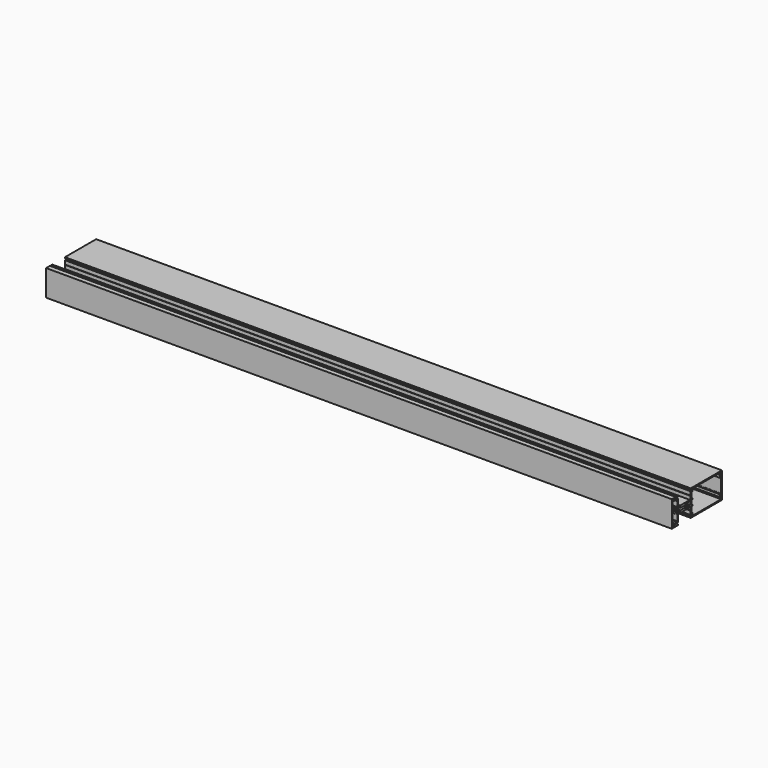
from build123d import *

# Parameters (mm, degrees)
F1_DEPTH = 1524
F2_DEPTH = 127


# Not quite as in the source:
# - ends of sketch curves that miss each other by under 0.0002 mm in the source are joined


with BuildPart() as f1:
    # F0 (on Right) → F1 (new body)
    with BuildSketch(Plane.YZ):
        with BuildLine():
            Line((-18.542, -31.745936), (76.2, -31.745936))
            Line((76.2, -31.745936), (76.2, -31.263336))
            Line((76.2, -31.263336), (76.2, 31.754064))
            Line((76.2, 31.754064), (-18.542, 31.754064))
            ThreePointArc((-18.542, 31.754064), (-18.9012102448, 31.6052742448), (-19.05, 31.246064))
            Line((-19.05, 31.246064), (-19.05, 29.163264))
            ThreePointArc((-19.05, 29.163264), (-18.8142131165, 28.8110223914), (-18.3986921218, 28.894759529))
            ThreePointArc((-18.3986921218, 28.894759529), (-17.6552092218, 29.3942029198), (-16.7769032, 29.569664))
            Line((-16.7769032, 29.569664), (-16.51, 29.569664))
            ThreePointArc((-16.51, 29.569664), (-15.6119743879, 29.1976896121), (-15.24, 28.299664))
            Line((-15.24, 28.299664), (-15.24, 26.064464))
            ThreePointArc((-15.24, 26.064464), (-15.6119743879, 25.1664383879), (-16.51, 24.794464))
            Line((-16.51, 24.794464), (-16.7769032, 24.794464))
            ThreePointArc((-16.7769032, 24.794464), (-17.6552092218, 24.9699250802), (-18.3986871392, 25.4693734208))
            ThreePointArc((-18.3986871392, 25.4693734208), (-18.8142131165, 25.5531056086), (-19.05, 25.200864))
            Line((-19.05, 25.200864), (-19.05, 17.466564))
            Line((-19.05, 17.466564), (-19.05, 16.260064))
            Line((-19.05, 16.260064), (-18.669, 15.879064))
            Line((-18.669, 15.879064), (-19.05, 15.498064))
            Line((-19.05, 15.498064), (-19.05, 6.684264))
            ThreePointArc((-19.05, 6.684264), (-19.1243948776, 6.5046588776), (-19.304, 6.430264))
            Line((-19.304, 6.430264), (-20.7264, 6.430264))
            ThreePointArc((-20.7264, 6.430264), (-20.9060051224, 6.5046588776), (-20.9804, 6.684264))
            Line((-20.9804, 6.684264), (-20.9804, 7.700264))
            ThreePointArc((-20.9804, 7.700264), (-21.0547948776, 7.8798691224), (-21.2344, 7.954264))
            Line((-21.2344, 7.954264), (-22.225, 7.954264))
            Line((-22.225, 7.954264), (-31.75, 7.954264))
            Line((-31.75, 7.954264), (-41.275, 7.954264))
            Line((-41.275, 7.954264), (-50.8, 7.954264))
            Line((-50.8, 7.954264), (-50.8, 6.938264))
            Line((-50.8, 6.938264), (-51.181, 6.557264))
            Line((-51.181, 6.557264), (-50.8, 6.176264))
            Line((-50.8, 6.176264), (-50.8, 4.322064))
            Line((-50.8, 4.322064), (-51.181, 3.941064))
            Line((-51.181, 3.941064), (-50.8, 3.560064))
            Line((-50.8, 3.560064), (-50.8, 2.544064))
            Line((-50.8, 2.544064), (-39.878, 2.544064))
            Line((-39.878, 2.544064), (-34.3379298, 1.0596118))
            ThreePointArc((-34.3379298, 1.0596118), (-33.528, 0.004064), (-34.337931039, -1.0514791763))
            Line((-34.337931039, -1.0514791763), (-39.878, -2.535936))
            Line((-39.878, -2.535936), (-50.8, -2.535936))
            Line((-50.8, -2.535936), (-50.8, -3.551936))
            Line((-50.8, -3.551936), (-51.181, -3.932936))
            Line((-51.181, -3.932936), (-50.8, -4.313936))
            Line((-50.8, -4.313936), (-50.8, -6.168136))
            Line((-50.8, -6.168136), (-51.181, -6.549136))
            Line((-51.181, -6.549136), (-50.8, -6.930136))
            Line((-50.8, -6.930136), (-50.8, -7.946136))
            Line((-50.8, -7.946136), (-21.2344, -7.946136))
            ThreePointArc((-21.2344, -7.946136), (-21.0547948776, -7.8717411224), (-20.9804, -7.692136))
            Line((-20.9804, -7.692136), (-20.9804, -6.676136))
            ThreePointArc((-20.9804, -6.676136), (-20.9060051224, -6.4965308776), (-20.7264, -6.422136))
            Line((-20.7264, -6.422136), (-19.304, -6.422136))
            ThreePointArc((-19.304, -6.422136), (-19.1243948776, -6.4965308776), (-19.05, -6.676136))
            Line((-19.05, -6.676136), (-19.05, -10.308336))
            Line((-19.05, -10.308336), (-19.05, -15.489936))
            Line((-19.05, -15.489936), (-18.669, -15.870936))
            Line((-18.669, -15.870936), (-19.05, -16.251936))
            Line((-19.05, -16.251936), (-19.05, -21.433536))
            Line((-19.05, -21.433536), (-19.05, -25.192736))
            ThreePointArc((-19.05, -25.192736), (-18.8142131165, -25.5449776086), (-18.3986921218, -25.461240471))
            ThreePointArc((-18.3986921218, -25.461240471), (-17.6552092218, -24.9617970802), (-16.7769032, -24.786336))
            Line((-16.7769032, -24.786336), (-16.51, -24.786336))
            ThreePointArc((-16.51, -24.786336), (-15.6119743879, -25.1583103879), (-15.24, -26.056336))
            Line((-15.24, -26.056336), (-15.24, -28.291536))
            ThreePointArc((-15.24, -28.291536), (-15.6119743879, -29.1895616121), (-16.51, -29.561536))
            Line((-16.51, -29.561536), (-16.7769032, -29.561536))
            ThreePointArc((-16.7769032, -29.561536), (-17.6552092218, -29.3860749198), (-18.3986871392, -28.8866265792))
            ThreePointArc((-18.3986871392, -28.8866265792), (-18.8142131165, -28.8028943914), (-19.05, -29.155136))
            Line((-19.05, -29.155136), (-19.05, -31.237936))
            ThreePointArc((-19.05, -31.237936), (-18.9012102448, -31.5971462448), (-18.542, -31.745936))
        make_face()
        with BuildLine():
            Line((-34.9879412, 5.414264), (-23.2150666, 5.414264))
            ThreePointArc((-23.2150666, 5.414264), (-22.1855160091, 4.3015310162), (-20.7264, 3.890264))
            Line((-20.7264, 3.890264), (-19.05, 3.890264))
            Line((-19.05, 3.890264), (-19.05, -3.882136))
            Line((-19.05, -3.882136), (-20.7264, -3.882136))
            ThreePointArc((-20.7264, -3.882136), (-22.1855160091, -4.2934030162), (-23.2150784839, -5.4061299355))
            Line((-23.2150784839, -5.4061299355), (-34.9879412, -5.406136))
            ThreePointArc((-34.9879412, -5.406136), (-35.7434215946, -4.7436014378), (-35.1851700405, -3.9081028591))
            Line((-35.1851700405, -3.9081028591), (-33.6805524, -3.504946))
            ThreePointArc((-33.6805524, -3.504946), (-30.988, 0.004064), (-33.6805547502, 3.513065229))
            Line((-33.6805547502, 3.513065229), (-35.1851722, 3.9162228))
            ThreePointArc((-35.1851722, 3.9162228), (-35.7434215946, 4.7517294378), (-34.9879412, 5.414264))
        make_face(mode=Mode.SUBTRACT)
        with BuildLine():
            Line((-16.51, 5.922264), (-13.208, 5.922264))
            ThreePointArc((-13.208, 5.922264), (-12.8487897552, 6.0710537552), (-12.7, 6.430264))
            Line((-12.7, 6.430264), (-12.7, 7.446264))
            ThreePointArc((-12.7, 7.446264), (-12.8487897552, 7.8054742448), (-13.208, 7.954264))
            Line((-13.208, 7.954264), (-15.875, 7.954264))
            Line((-15.875, 7.954264), (-15.875, 22.737064))
            Line((-15.875, 22.737064), (-13.208, 22.737064))
            ThreePointArc((-13.208, 22.737064), (-12.8487897552, 22.8858537552), (-12.7, 23.245064))
            Line((-12.7, 23.245064), (-12.7, 28.452064))
            ThreePointArc((-12.7, 28.452064), (-12.4768153673, 28.9908793673), (-11.938, 29.214064))
            Line((-11.938, 29.214064), (73.66, 29.214064))
            Line((73.66, 29.214064), (73.66, 25.150064))
            ThreePointArc((73.66, 25.150064), (73.2136307345, 24.0724332655), (72.136, 23.626064))
            Line((72.136, 23.626064), (70.612, 23.626064))
            Line((70.612, 23.626064), (70.612, 17.657064))
            Line((70.612, 17.657064), (72.136, 17.657064))
            ThreePointArc((72.136, 17.657064), (73.2136307345, 17.2106947345), (73.66, 16.133064))
            Line((73.66, 16.133064), (73.66, -16.124936))
            ThreePointArc((73.66, -16.124936), (73.2136307345, -17.2025667345), (72.136, -17.648936))
            Line((72.136, -17.648936), (70.612, -17.648936))
            Line((70.612, -17.648936), (70.612, -23.617936))
            Line((70.612, -23.617936), (72.136, -23.617936))
            ThreePointArc((72.136, -23.617936), (73.2136307345, -24.0643052655), (73.66, -25.141936))
            Line((73.66, -25.141936), (73.66, -29.205936))
            Line((73.66, -29.205936), (-11.938, -29.205936))
            ThreePointArc((-11.938, -29.205936), (-12.4768153673, -28.9827513673), (-12.7, -28.443936))
            Line((-12.7, -28.443936), (-12.7, -23.236936))
            ThreePointArc((-12.7, -23.236936), (-12.8487897552, -22.8777257552), (-13.208, -22.728936))
            Line((-13.208, -22.728936), (-15.875, -22.728936))
            Line((-15.875, -22.728936), (-15.875, -7.946136))
            Line((-15.875, -7.946136), (-13.208, -7.946136))
            ThreePointArc((-13.208, -7.946136), (-12.8487897552, -7.7973462448), (-12.7, -7.438136))
            Line((-12.7, -7.438136), (-12.7, -6.422136))
            ThreePointArc((-12.7, -6.422136), (-12.8487897552, -6.0629257552), (-13.208, -5.914136))
            Line((-13.208, -5.914136), (-16.51, -5.914136))
            Line((-16.51, -5.914136), (-16.51, 5.922264))
        make_face(mode=Mode.SUBTRACT)
    extrude(amount=F1_DEPTH)


with BuildPart() as f1b:
    # F0 (on Right) → F1, piece 2 (new body)
    with BuildSketch(Plane.YZ):
        with BuildLine():
            Line((-57.15, 6.366764), (-57.15, 7.954264))
            Line((-57.15, 7.954264), (-57.15, 25.200864))
            ThreePointArc((-57.15, 25.200864), (-57.3857786086, 25.5531021971), (-57.8012952623, 25.4693811711))
            ThreePointArc((-57.8012952623, 25.4693811711), (-58.5447653782, 24.9699250802), (-59.4230714, 24.794464))
            Line((-59.4230714, 24.794464), (-59.69, 24.794464))
            ThreePointArc((-59.69, 24.794464), (-60.5880256121, 25.1664383879), (-60.96, 26.064464))
            Line((-60.96, 26.064464), (-60.96, 28.299664))
            ThreePointArc((-60.96, 28.299664), (-60.5880256121, 29.1976896121), (-59.69, 29.569664))
            Line((-59.69, 29.569664), (-59.4230714, 29.569664))
            ThreePointArc((-59.4230714, 29.569664), (-58.5447653782, 29.3942029198), (-57.8012874608, 28.8947545792))
            ThreePointArc((-57.8012874608, 28.8947545792), (-57.3857786086, 28.8110258029), (-57.15, 29.163264))
            Line((-57.15, 29.163264), (-57.15, 31.246064))
            ThreePointArc((-57.15, 31.246064), (-57.2987897552, 31.6052742448), (-57.658, 31.754064))
            Line((-57.658, 31.754064), (-62.3824, 31.754064))
            ThreePointArc((-62.3824, 31.754064), (-62.9212153673, 31.5308793673), (-63.1444, 30.992064))
            Line((-63.1444, 30.992064), (-63.1444, 29.976064))
            ThreePointArc((-63.1444, 29.976064), (-63.5163743879, 29.0780383879), (-64.4144, 28.706064))
            ThreePointArc((-64.4144, 28.706064), (-65.1549312963, 28.9443114138), (-65.6176205987, 29.5696649462))
            Line((-65.6176205987, 29.5696649462), (-70.2564, 26.8914626))
            ThreePointArc((-70.2564, 26.8914626), (-70.6282817077, 25.5035810224), (-69.2403998224, 25.1316994923))
            Line((-69.2403998224, 25.1316994923), (-66.5689296, 26.674064))
            Line((-66.5689296, 26.674064), (-63.1444, 26.674064))
            Line((-63.1444, 26.674064), (-63.1444, 23.778464))
            ThreePointArc((-63.1444, 23.778464), (-62.6980307345, 22.7008332655), (-61.6204, 22.254464))
            Line((-61.6204, 22.254464), (-59.69, 22.254464))
            Line((-59.69, 22.254464), (-59.69, 8.259064))
            Line((-59.69, 8.259064), (-60.325, 7.624064))
            Line((-60.325, 7.624064), (-60.325, 6.354064))
            Line((-60.325, 6.354064), (-60.325, 3.382264))
            Line((-60.325, 3.382264), (-57.15, 3.382264))
            Line((-57.15, 3.382264), (-57.15, 4.957064))
            Line((-57.15, 4.957064), (-56.769, 5.338064))
            Line((-56.769, 5.338064), (-57.15, 5.719064))
            Line((-57.15, 5.719064), (-57.15, 6.366764))
        make_face()
    extrude(amount=F1_DEPTH)


with BuildPart() as f1c:
    # F0 (on Right) → F1, piece 3 (new body)
    with BuildSketch(Plane.YZ):
        with BuildLine():
            ThreePointArc((-65.4304, 29.722064), (-65.1328204897, 29.0036435103), (-64.4144, 28.706064))
            ThreePointArc((-64.4144, 28.706064), (-63.6959795103, 29.0036435103), (-63.3984, 29.722064))
            Line((-63.3984, 29.722064), (-63.3984, 30.230064))
            ThreePointArc((-63.3984, 30.230064), (-63.8447692655, 31.3076947345), (-64.9224, 31.754064))
            Line((-64.9224, 31.754064), (-76.2, 31.754064))
            Line((-76.2, 31.754064), (-76.2, -31.745936))
            Line((-76.2, -31.745936), (-64.9224, -31.745936))
            ThreePointArc((-64.9224, -31.745936), (-63.8447692655, -31.2995667345), (-63.3984, -30.221936))
            Line((-63.3984, -30.221936), (-63.3984, -29.713936))
            ThreePointArc((-63.3984, -29.713936), (-63.6959795103, -28.9955155103), (-64.4144, -28.697936))
            ThreePointArc((-64.4144, -28.697936), (-65.1328204897, -28.9955155103), (-65.4304, -29.713936))
            Line((-65.4304, -29.713936), (-65.4304, -30.475936))
            Line((-65.4304, -30.475936), (-74.676, -30.475936))
            Line((-74.676, -30.475936), (-74.676, 30.484064))
            Line((-74.676, 30.484064), (-65.4304, 30.484064))
            Line((-65.4304, 30.484064), (-65.4304, 29.722064))
        make_face()
    extrude(amount=F1_DEPTH)


with BuildPart() as f1d:
    # F0 (on Right) → F1, piece 4 (new body)
    with BuildSketch(Plane.YZ):
        with BuildLine():
            Line((-57.15, -25.192736), (-57.15, -7.946136))
            Line((-57.15, -7.946136), (-57.15, -6.358636))
            Line((-57.15, -6.358636), (-57.15, -5.710936))
            Line((-57.15, -5.710936), (-56.769, -5.329936))
            Line((-56.769, -5.329936), (-57.15, -4.948936))
            Line((-57.15, -4.948936), (-57.15, -3.374136))
            Line((-57.15, -3.374136), (-60.325, -3.374136))
            Line((-60.325, -3.374136), (-60.325, -6.345936))
            Line((-60.325, -6.345936), (-60.325, -7.615936))
            Line((-60.325, -7.615936), (-59.69, -8.250936))
            Line((-59.69, -8.250936), (-59.69, -22.246336))
            Line((-59.69, -22.246336), (-61.6204, -22.246336))
            ThreePointArc((-61.6204, -22.246336), (-62.6980307345, -22.6927052655), (-63.1444, -23.770336))
            Line((-63.1444, -23.770336), (-63.1444, -26.665936))
            Line((-63.1444, -26.665936), (-66.5689296, -26.665936))
            Line((-66.5689296, -26.665936), (-69.2404, -25.1235718))
            ThreePointArc((-69.2404, -25.1235718), (-70.6282817077, -25.4954530224), (-70.2564001776, -26.8833349077))
            Line((-70.2564001776, -26.8833349077), (-65.6176234, -29.561536))
            ThreePointArc((-65.6176234, -29.561536), (-65.1549312963, -28.9361834138), (-64.4144, -28.697936))
            ThreePointArc((-64.4144, -28.697936), (-63.5163743879, -29.0699103879), (-63.1444, -29.967936))
            Line((-63.1444, -29.967936), (-63.1444, -30.983936))
            ThreePointArc((-63.1444, -30.983936), (-62.9212153673, -31.5227513673), (-62.3824, -31.745936))
            Line((-62.3824, -31.745936), (-57.658, -31.745936))
            ThreePointArc((-57.658, -31.745936), (-57.2987897552, -31.5971462448), (-57.15, -31.237936))
            Line((-57.15, -31.237936), (-57.15, -29.155136))
            ThreePointArc((-57.15, -29.155136), (-57.3857786086, -28.8028978029), (-57.8012952623, -28.8866188289))
            ThreePointArc((-57.8012952623, -28.8866188289), (-58.5447653782, -29.3860749198), (-59.4230714, -29.561536))
            Line((-59.4230714, -29.561536), (-59.69, -29.561536))
            ThreePointArc((-59.69, -29.561536), (-60.5880256121, -29.1895616121), (-60.96, -28.291536))
            Line((-60.96, -28.291536), (-60.96, -26.056336))
            ThreePointArc((-60.96, -26.056336), (-60.5880256121, -25.1583103879), (-59.69, -24.786336))
            Line((-59.69, -24.786336), (-59.4230714, -24.786336))
            ThreePointArc((-59.4230714, -24.786336), (-58.5447653782, -24.9617970802), (-57.8012874608, -25.4612454208))
            ThreePointArc((-57.8012874608, -25.4612454208), (-57.3857786086, -25.5449741971), (-57.15, -25.192736))
        make_face()
    extrude(amount=F1_DEPTH)


with BuildPart() as f2:
    # F0 (on Right) → F2 (new body)
    with BuildSketch(Plane.YZ):
        Polygon((-57.15, -3.374136), (-57.15, 3.382264), (-60.325, 3.382264), (-60.325, 0.385064), (-59.944, 0.004064), (-60.325, -0.376936), (-60.325, -3.374136), align=None)
    extrude(amount=F2_DEPTH)


solid = Compound([f1.part, f1b.part, f1c.part, f1d.part, f2.part])
